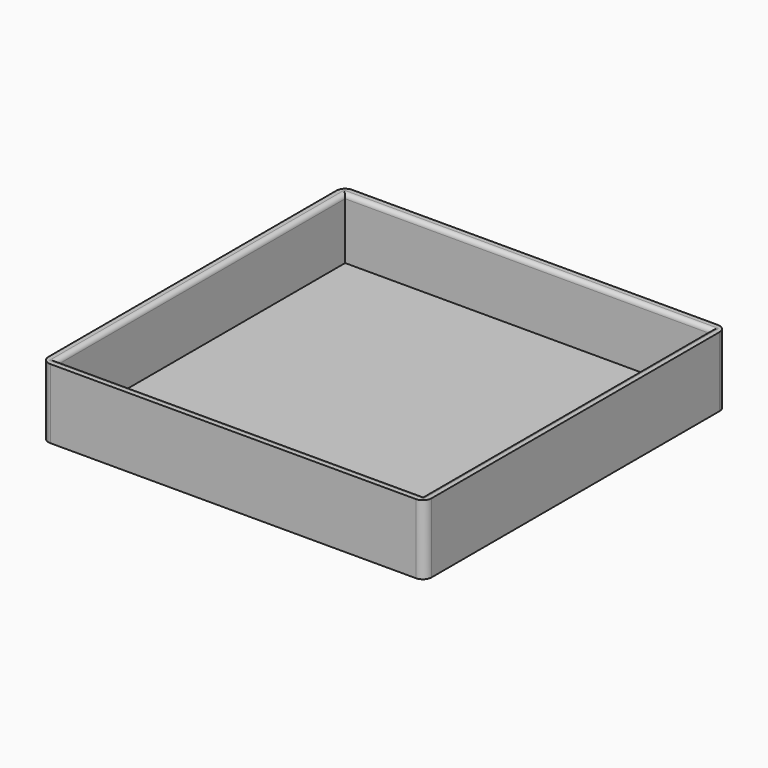
from build123d import *

# Parameters (mm, degrees)
F1_DEPTH = 4
F2_T     = 0.5
F3_R     = 0.25


# Not quite as in the source:
# - a shell that OpenCascade refuses in one call is made with other operations: the cavity is built on its own and cut out


with BuildPart() as f1:
    # F0 (on Top) → F1 (new body)
    with BuildSketch(Plane.XY):
        with BuildLine():
            Line((10.5, 10.835), (-10.5, 10.835))
            ThreePointArc((-10.5, 10.835), (-10.8535533906, 10.6885533906), (-11, 10.335))
            Line((-11, 10.335), (-11, -10.335))
            ThreePointArc((-11, -10.335), (-10.8535533906, -10.6885533906), (-10.5, -10.835))
            Line((-10.5, -10.835), (10.5, -10.835))
            ThreePointArc((10.5, -10.835), (10.8535533906, -10.6885533906), (11, -10.335))
            Line((11, -10.335), (11, 10.335))
            ThreePointArc((11, 10.335), (10.8535533906, 10.6885533906), (10.5, 10.835))
        make_face()
    extrude(amount=F1_DEPTH)

    # F2: shell of thickness 0.5, made by hand


with BuildPart() as f2_core1:
    # F2_t2: copy of F1
    add(f1.part)

    # the walls: a layer under each face that stays
    f2_faces = [f2_core1.faces().sort_by_distance(p)[0] for p in [
        (0, 10.835, 2),
        (-11, 0, 2),
        (0, -10.835, 2),
        (11, 0, 2),
        (0, 0, 0),
    ]]
    thicken(f2_faces, amount=-F2_T, mode=Mode.SUBTRACT)


with BuildPart() as f1_1:
    add(f1.part)

    # what is left inside the walls is the cavity
    f2_cavity = [f2_core1.part.solids().sort_by_distance(p)[0] for p in [
        (0, -3.445, 0.505),
    ]]
    add(f2_cavity, mode=Mode.SUBTRACT)

    # F3
    f3_edges = [f1_1.edges().sort_by_distance(p)[0] for p in [
        (10.5, 0, 4),
        (0, 10.335, 4),
        (-10.5, 0, 4),
        (0, -10.335, 4),
    ]]
    fillet(f3_edges, radius=F3_R)


solid = f1_1.part
